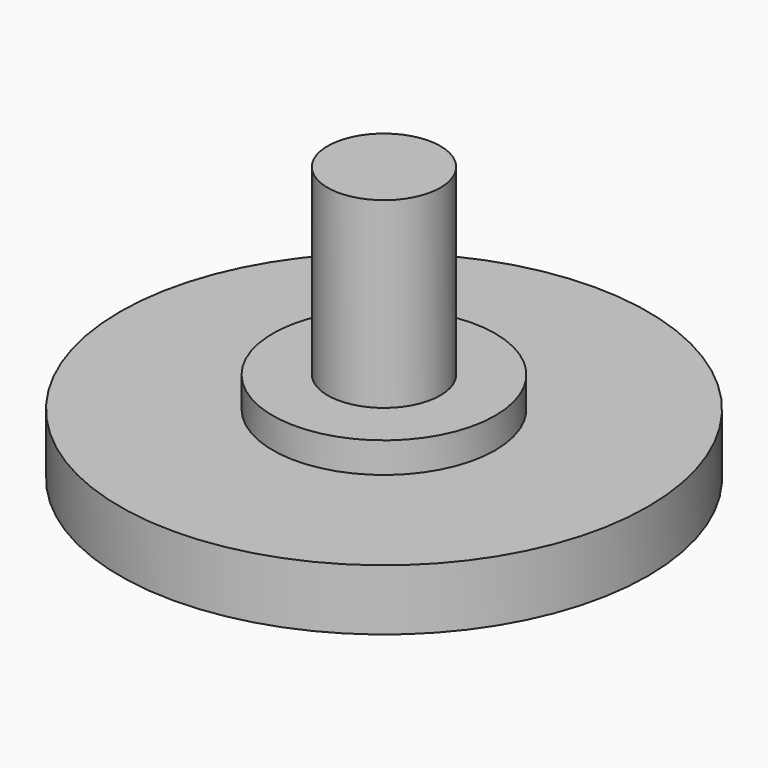
from build123d import *

# Parameters (mm, degrees)
F0_R     = 2.35
F1_DEPTH = 11.43
F0_R_2   = 4.636
F2_DEPTH = 3.81
F0_R_3   = 11
F3_DEPTH = 2.54
F5_DEPTH = 1.27
F6_SIZE  = 1.26999
F7_R     = 1.26999


# Not quite as in the source:
# - a fillet or chamfer is up to 0.001 mm smaller than in the source, because OpenCascade refuses the exact size


with BuildPart() as f1:
    # F0 (on Top) → F1 (new body)
    with BuildSketch(Plane.XY):
        Circle(F0_R)
    extrude(amount=F1_DEPTH)

    # F0 (on Top) → F2 (join)
    with BuildSketch(Plane.XY):
        Circle(F0_R_2)
        Circle(F0_R, mode=Mode.SUBTRACT)
    extrude(amount=F2_DEPTH)

    # F0 (on Top) → F3 (join)
    with BuildSketch(Plane.XY):
        Circle(F0_R_3)
        Circle(F0_R_2, mode=Mode.SUBTRACT)
    extrude(amount=F3_DEPTH)

    # F4 (on face) → F5 (join)
    with BuildSketch(Plane.XY):
        with BuildLine():
            ThreePointArc((0, 5.4110168739), (3.4329052601, -0.1769831261), (0, -5.7649831261))
            Line((0, -5.7649831261), (0, -9.0669831261))
            ThreePointArc((0, -9.0669831261), (6.8902932862, -0.1769831261), (0, 8.7130168739))
            Line((0, 8.7130168739), (0, 5.4110168739))
        make_face()
        Polygon((0, -9.0669831261), (0, -5.7649831261), (0, 5.4110168739), (0, 8.7130168739), (-3.302, 8.7130168739), (-3.302, -9.0669831261), align=None)
    extrude(amount=-F5_DEPTH)

    # F6 (size 1.27 in the source; OpenCascade refuses exactly that, so slightly less here)
    f6_edges = [f1.edges().sort_by_distance(p)[0] for p in [
        (-3.302, -0.176983, -1.27),
        (0, -0.176983, -1.27),
    ]]
    chamfer(f6_edges, length=F6_SIZE)

    # F7 (radius 1.27 in the source; OpenCascade refuses exactly that, so slightly less here)
    f7_edges = [f1.edges().sort_by_distance(p)[0] for p in [
        (6.890293, -0.176983, -1.27),
    ]]
    fillet(f7_edges, radius=F7_R)


solid = f1.part
